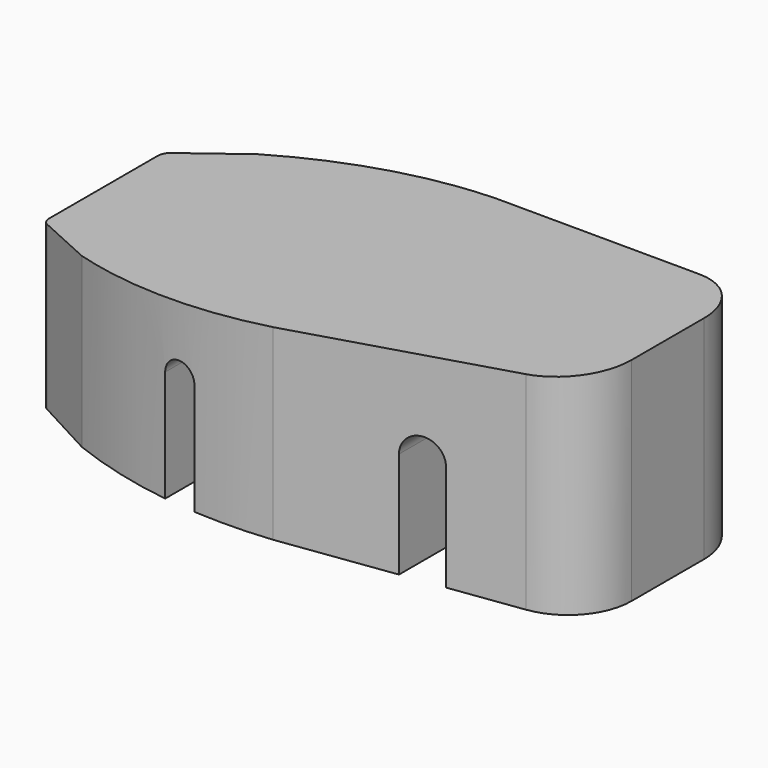
from build123d import *

# Parameters (mm, degrees)
F1_DEPTH = 200
F3_DEPTH = 150
F4_W     = 40
F4_H     = 120
F4_W_2   = 30
F5_DEPTH = 150
F6_R     = 19.99999
F7_R     = 15
F7_R_2   = 14.99999


# Not quite as in the source:
# - a fillet or chamfer is up to 0.001 mm smaller than in the source, because OpenCascade refuses the exact size
# - ends of sketch curves that miss each other by under 0.0002 mm in the source are joined


with BuildPart() as f1:
    # F0 (on Top) → F1 (new body)
    with BuildSketch(Plane.XY):
        with BuildLine():
            Line((-203.32088, 103.750296), (-260.740998, 72.83177))
            ThreePointArc((-260.740998, 72.83177), (-264.5851610502, 69.1549250028), (-266, 64.027059))
            Line((-266, 64.027059), (-266, -64.027059))
            ThreePointArc((-266, -64.027059), (-264.5851610502, -69.1549250028), (-260.7409980515, -72.8317700956))
            Line((-260.7409980515, -72.8317700956), (-203.32088, -103.750296))
            ThreePointArc((-203.32088, -103.750296), (-103.8608632236, -129.7071209998), (-1.082674041, -131.348924606))
            Line((-1.082674041, -131.348924606), (214.09118, -102.064591))
            ThreePointArc((214.09118, -102.064591), (251.1966304028, -82.0748460353), (266, -42.612654))
            Line((266, -42.612654), (266, 42.612654))
            ThreePointArc((266, 42.612654), (251.1966304028, 82.0748460353), (214.0911799923, 102.0645909435))
            Line((214.0911799923, 102.0645909435), (-1.082674, 131.348925))
            ThreePointArc((-1.082674, 131.348925), (-103.8608632236, 129.7071209998), (-203.32088, 103.750296))
        make_face()
    extrude(amount=F1_DEPTH)

    # F2 (on Front) → F3 (cut, symmetric)
    with BuildSketch(Plane.XZ):
        Polygon((266, 200), (-266, 200), (-266, 153), align=None)
    extrude(amount=F3_DEPTH, both=True, mode=Mode.SUBTRACT)

    # F4 (on Front) → F5 (cut, symmetric)
    with BuildSketch(Plane.XZ):
        with Locations((126, 60)):
            Rectangle(F4_W, F4_H)
        with Locations((-89, 60)):
            Rectangle(F4_W_2, F4_H)
    extrude(amount=F5_DEPTH, both=True, mode=Mode.SUBTRACT)

    # F6 (radius 20 in the source; OpenCascade refuses exactly that, so slightly less here)
    f6_edges = [f1.edges().sort_by_distance(p)[0] for p in [
        (146, 0, 120),
        (106, 0, 120),
    ]]
    fillet(f6_edges, radius=F6_R)

    # F7 (call 1 of 2: OpenCascade refuses the feature's edges together)
    f7_edges = [f1.edges().sort_by_distance(p)[0] for p in [
        (-74, 0, 120),
    ]]
    fillet(f7_edges, radius=F7_R)

    # F7#2 (call 2 of 2) (radius 15 in the source; OpenCascade refuses exactly that, so slightly less here)
    f7_2_edges = [f1.edges().sort_by_distance(p)[0] for p in [
        (-104, 0, 120),
    ]]
    fillet(f7_2_edges, radius=F7_R_2)


solid = f1.part
